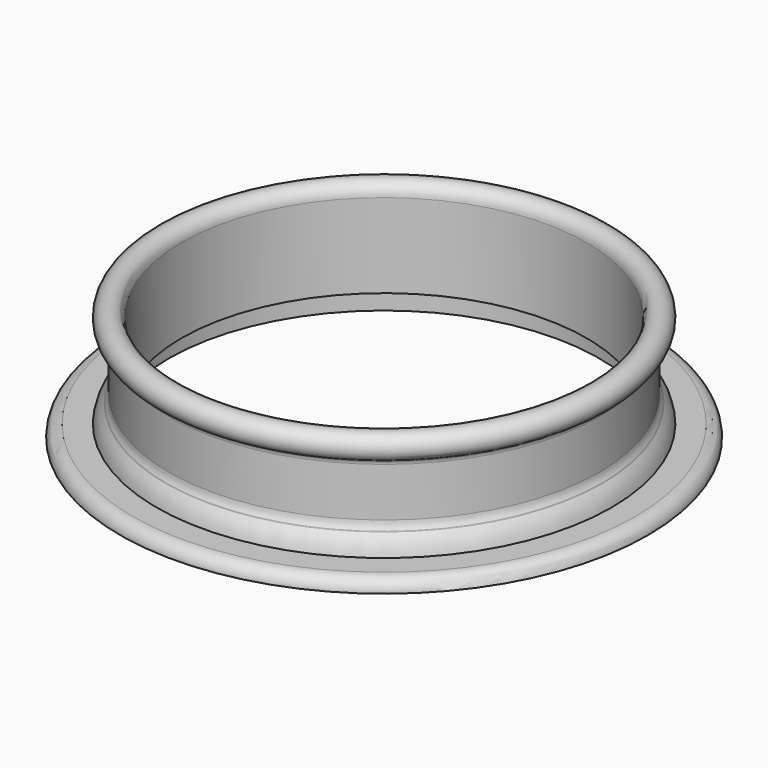
from build123d import *

# Parameters (mm, degrees)
F0_R      = 42
F0_R_2    = 36.5
F1_DEPTH  = 2
F4_R      = 42
F5_DEPTH  = 1
F6_R      = 34.5
F6_R_2    = 32.5
F7_DEPTH  = 3
F8_R      = 42.35
F8_R_2    = 42
F9_DEPTH  = 2
F10_R     = 1.99999
F11_R     = 32.5
F12_DEPTH = 25
F13_R     = 36.5
F13_R_2   = 32.5
F14_DEPTH = 5
F15_R     = 34.5
F16_DEPTH = 3.5
F17_R     = 1
F18_SIZE  = 1.5


# Not quite as in the source:
# - a fillet or chamfer that OpenCascade refuses, or shapes differently, is made with other operations: its cross-section is extruded or revolved along the edge and cut away or added
# - a fillet or chamfer is up to 0.001 mm smaller than in the source, because OpenCascade refuses the exact size


with BuildPart() as f1:
    # F0 (on Top) → F1 (new body)
    with BuildSketch(Plane.XY):
        Circle(F0_R)
        Circle(F0_R_2, mode=Mode.SUBTRACT)
    extrude(amount=F1_DEPTH)

    # F2 (on Front) → F3 (revolve)
    with BuildSketch(Plane.XZ):
        with BuildLine():
            Line((36.5, 0), (36.5, 2))
            Line((36.5, 2), (35.5, 2))
            ThreePointArc((35.5, 2), (34.7928932188, 2.2928932188), (34.5, 3))
            Line((34.5, 3), (34.5, 14.1715728753))
            ThreePointArc((34.5, 14.1715728753), (34.6835034191, 14.7489231444), (35.1666666667, 15.1143819168))
            ThreePointArc((35.1666666667, 15.1143819168), (35.6547005384, 18.6329931619), (32.5, 17))
            Line((32.5, 17), (32.5, 2))
            ThreePointArc((32.5, 2), (33.0857864376, 0.5857864376), (34.5, 0))
            Line((34.5, 0), (36.5, 0))
        make_face()
    revolve(axis=Axis((0, 0, 63.5549128056), (0, 0, 1)))

    # F4 (on face) → F5 (join)
    with BuildSketch(Plane(origin=(0, 0, 0), x_dir=(1, 0, 0), z_dir=(0, 0, -1))):
        Circle(F4_R)
    extrude(amount=-F5_DEPTH)

    # F6 (on face) → F7 (join)
    with BuildSketch(Plane.XY.offset(1)):
        Circle(F6_R)
        Circle(F6_R_2, mode=Mode.SUBTRACT)
    extrude(amount=F7_DEPTH)

    # F8 (on face) → F9 (join)
    with BuildSketch(Plane.XY.offset(2)):
        Circle(F8_R)
        Circle(F8_R_2, mode=Mode.SUBTRACT)
    extrude(amount=-F9_DEPTH)

    # F10 (radius 2 in the source; OpenCascade refuses exactly that, so slightly less here)
    f10_edges = [f1.edges().sort_by_distance(p)[0] for p in [
        (-42.35, 0, 2),
    ]]
    fillet(f10_edges, radius=F10_R)

    # F11 (on face) → F12 (cut)
    with BuildSketch(Plane(origin=(0, 0, 0), x_dir=(1, 0, 0), z_dir=(0, 0, -1))):
        Circle(F11_R)
    extrude(amount=-F12_DEPTH, mode=Mode.SUBTRACT)

    # F13 (on face) → F14 (join)
    with BuildSketch(Plane(origin=(0, 0, 0), x_dir=(1, 0, 0), z_dir=(0, 0, -1))):
        Circle(F13_R)
        Circle(F13_R_2, mode=Mode.SUBTRACT)
    extrude(amount=-F14_DEPTH)

    # F15 (on face) → F16 (cut)
    with BuildSketch(Plane(origin=(0, 0, 0), x_dir=(1, 0, 0), z_dir=(0, 0, -1))):
        Circle(F15_R)
    extrude(amount=-F16_DEPTH, mode=Mode.SUBTRACT)

    # F17
    f17_edges = [f1.edges().sort_by_distance(p)[0] for p in [
        (-34.5, 0, 3.5),
    ]]
    fillet(f17_edges, radius=F17_R)

    # F18
    f18_edges = [f1.edges().sort_by_distance(p)[0] for p in [
        (-36.5, 0, 5),
    ]]
    chamfer(f18_edges, length=F18_SIZE)

    # F19: fillet of radius 2 on 1 edges, made by hand

    # F19_s1 → F19_t2 (revolve)
    with BuildSketch(Plane.XZ):
        with BuildLine():
            ThreePointArc((35, 5), (34.6291713066, 5.6157688743), (34.5, 6.3228756555))
            Line((34.5, 6.3228756555), (34.5, 5))
            Line((34.5, 5), (35, 5))
        make_face()
    revolve(axis=Axis((0, 0, 5), (0, 0, 1)))

    # F20: fillet of radius 5 on 1 edges, made by hand

    # F20_s1 → F20_t2 (revolve, cut)
    with BuildSketch(Plane.XZ):
        with BuildLine():
            ThreePointArc((36.5, 2), (36.0313524106, 3.5831387774), (35.0726619787, 4.9273380213))
            Line((35.0726619787, 4.9273380213), (36.5, 3.5))
            Line((36.5, 3.5), (36.5, 2))
        make_face()
    revolve(axis=Axis((0, 0, 3.5), (0, 0, -1)), mode=Mode.SUBTRACT)


solid = f1.part
